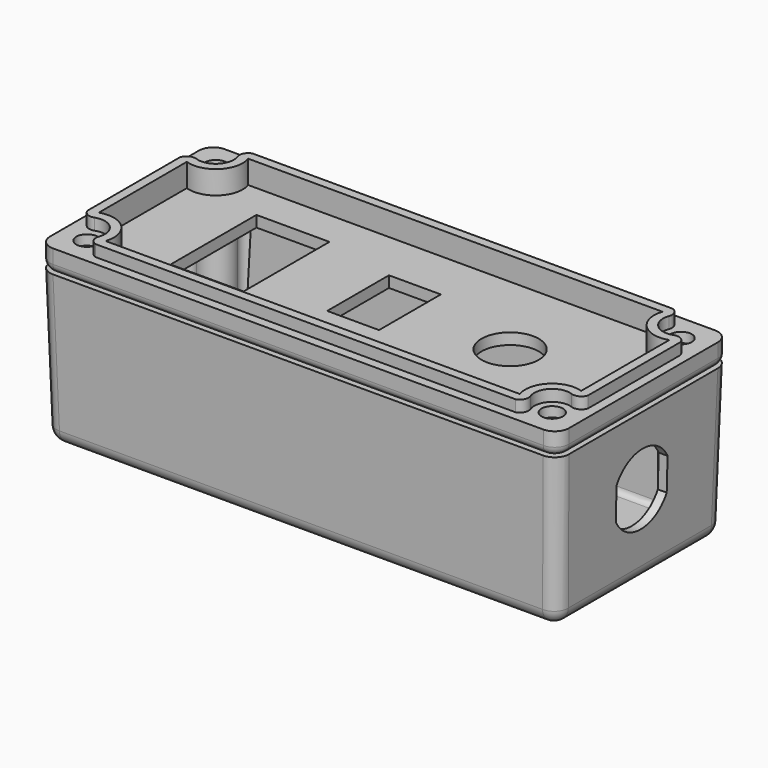
from build123d import *

# Parameters (mm, degrees)
F0_W            = 92.075
F0_H            = 38.1
F1_DEPTH        = 26.9748
F1_TAPER        = 1.5
F2_R            = 2.54
F3_T            = 1.5748
F6_DEPTH        = 23.0124
F8_D            = 2.7051
F8_DEPTH        = 12.7
F8_TIP          = 0.8126940303
F10_DEPTH       = 4.064
F13_DEPTH       = 2.032
F15_DEPTH       = 2.0828
F17_D           = 3.7973
F17_CSINK_D     = 7.7978
F17_CSINK_ANGLE = 82
F18_T1_DEPTH    = 86.995
F18_T3_DEPTH    = 33.02
F18_T6_ANGLE    = 90
F18_T8_ANGLE    = 90
F18_T10_ANGLE   = 90
F18_T12_ANGLE   = 90
F19_W           = 12.954
F19_H           = 19.05
F19_R           = 5.08
F19_W_2         = 9.2
F19_H_2         = 13.7
F20_DEPTH       = 6.097
F22_DEPTH       = 92.0760001
F24_D           = 2.7051
F24_DEPTH       = 12.7
F24_TIP         = 0.8126940303


# Not quite as in the source:
# - a fillet or chamfer that OpenCascade refuses, or shapes differently, is made with other operations: its cross-section is extruded or revolved along the edge and cut away or added
# - a shell that OpenCascade refuses in one call is made with other operations: the cavity is built on its own and cut out


with BuildPart() as f1:
    # F0 (on Top) → F1 (new body)
    with BuildSketch(Plane.XY):
        with Locations((46.0375, 19.05)):
            Rectangle(F0_W, F0_H)
    extrude(amount=-F1_DEPTH, taper=F1_TAPER)

    # F2
    f2_edges = [f1.edges().sort_by_distance(p)[0] for p in [
        (91.72182, 0.35318, -13.4874),
        (46.0375, 0.70636, -26.9748),
        (0.35318, 0.35318, -13.4874),
        (0.35318, 37.74682, -13.4874),
        (0.70636, 19.05, -26.9748),
        (91.36864, 19.05, -26.9748),
        (91.72182, 37.74682, -13.4874),
        (46.0375, 37.39364, -26.9748),
    ]]
    fillet(f2_edges, radius=F2_R)

    # F3: shell of thickness 1.5748, made by hand


with BuildPart() as f3_core1:
    # F3_t2: copy of F1
    add(f1.part)

    # the walls: a layer under each face that stays
    f3_faces = [f3_core1.faces().sort_by_distance(p)[0] for p in [
        (0.3207944219, 19.05, -12.2506447244),
        (1.0647429252, 37.0352570748, -12.2643990402),
        (1.0647429252, 1.0647429252, -12.2643990402),
        (1.4083306813, 19.05, -26.2542069363),
        (46.0375, 37.7792055781, -12.2506447244),
        (46.0375, 0.3207944219, -12.2506447244),
        (91.0102570748, 37.0352570748, -12.2643990402),
        (91.0102570748, 1.0647429252, -12.2643990402),
        (91.7542055781, 19.05, -12.2506447244),
        (1.9274510394, 36.1725489858, -26.2542069186),
        (1.418333, 1.9278747208, -25.7674590413),
        (46.0375, 19.05, -26.9748),
        (46.0375, 36.6916693187, -26.2542069363),
        (46.0375, 1.4083306813, -26.2542069363),
        (90.1471252549, 36.6816670172, -25.7674590413),
        (90.1475489611, 1.9274510396, -26.2542069358),
        (90.6666693187, 19.05, -26.2542069363),
    ]]
    thicken(f3_faces, amount=-F3_T, mode=Mode.SUBTRACT)


with BuildPart() as f1_1:
    add(f1.part)

    # what is left inside the walls is the cavity
    f3_cavity = [f3_core1.part.solids().sort_by_distance(p)[0] for p in [
        (50.224462, 29.168476, -0.015748),
    ]]
    add(f3_cavity, mode=Mode.SUBTRACT)

    # F5 (on offset) → F6 (join, through all)
    with BuildSketch(Plane.XY.offset(-2.3876)):
        with BuildLine():
            ThreePointArc((1.5753398296, 28.8697382874), (2.2451150935, 30.1585071832), (3.6847191374, 30.351028267))
            ThreePointArc((3.6847191374, 30.351028267), (7.0075640303, 31.0924359697), (7.748971733, 34.4152808626))
            ThreePointArc((7.748971733, 34.4152808626), (7.9414928168, 35.8548849065), (9.2302617126, 36.5246601704))
            Line((9.2302617126, 36.5246601704), (1.5753398296, 36.5246601704))
            Line((1.5753398296, 36.5246601704), (1.5753398296, 28.8697382874))
        make_face()
        with BuildLine():
            Line((90.4996601704, 28.8697382874), (90.4996601704, 36.5246601704))
            Line((90.4996601704, 36.5246601704), (82.8447382874, 36.5246601704))
            ThreePointArc((82.8447382874, 36.5246601704), (84.1335071832, 35.8548849065), (84.326028267, 34.4152808626))
            ThreePointArc((84.326028267, 34.4152808626), (85.0674359697, 31.0924359697), (88.3902808626, 30.351028267))
            ThreePointArc((88.3902808626, 30.351028267), (89.8298849065, 30.1585071832), (90.4996601704, 28.8697382874))
        make_face()
        with BuildLine():
            ThreePointArc((7.748971733, 3.6847191374), (7.0075640303, 7.0075640303), (3.6847191374, 7.748971733))
            ThreePointArc((3.6847191374, 7.748971733), (2.2451150935, 7.9414928168), (1.5753398296, 9.2302617126))
            Line((1.5753398296, 9.2302617126), (1.5753398296, 1.5753398296))
            Line((1.5753398296, 1.5753398296), (9.2302617126, 1.5753398296))
            ThreePointArc((9.2302617126, 1.5753398296), (7.9414928168, 2.2451150935), (7.748971733, 3.6847191374))
        make_face()
        with BuildLine():
            Line((90.4996601704, 1.5753398296), (90.4996601704, 9.2302617126))
            ThreePointArc((90.4996601704, 9.2302617126), (89.8298849065, 7.9414928168), (88.3902808626, 7.748971733))
            ThreePointArc((88.3902808626, 7.748971733), (85.0674359697, 7.0075640303), (84.326028267, 3.6847191374))
            ThreePointArc((84.326028267, 3.6847191374), (84.1335071832, 2.2451150935), (82.8447382874, 1.5753398296))
            Line((82.8447382874, 1.5753398296), (90.4996601704, 1.5753398296))
        make_face()
    extrude(amount=-F6_DEPTH)

    # F8
    with Locations(Plane.XY.offset(-2.3876)):
        with Locations((4.7625, 33.3375), (4.7625, 4.7625), (87.3125, 4.7625), (87.3125, 33.3375)):
            Hole(F8_D / 2, depth=F8_DEPTH)
            with Locations((0, 0, -(F8_DEPTH + F8_TIP / 2))):  # 118° drill point
                Cone(0, F8_D / 2, F8_TIP, mode=Mode.SUBTRACT)

    # F21 (on Right) → F22 (cut, through all)
    with BuildSketch(Plane.YZ):
        with BuildLine():
            Line((24.7015, -15.1459940556), (24.7015, -9.3552953931))
            ThreePointArc((24.7015, -9.3552953931), (19.05, -5.9006447244), (13.3985, -9.3552953931))
            Line((13.3985, -9.3552953931), (13.3985, -15.1459940556))
            ThreePointArc((13.3985, -15.1459940556), (19.05, -18.6006447244), (24.7015, -15.1459940556))
        make_face()
    extrude(amount=F22_DEPTH, mode=Mode.SUBTRACT)

    # F24
    with Locations(Plane(origin=(0, 0, -26.9748), x_dir=(1, 0, 0), z_dir=(0, 0, -1))):
        with Locations((14.2875, -19.05), (77.7875, -19.05)):
            Hole(F24_D / 2, depth=F24_DEPTH)
            with Locations((0, 0, -(F24_DEPTH + F24_TIP / 2))):  # 118° drill point
                Cone(0, F24_D / 2, F24_TIP, mode=Mode.SUBTRACT)


with BuildPart() as f10:
    # F9 (on Top) → F10 (new body)
    with BuildSketch(Plane.XY):
        with BuildLine():
            ThreePointArc((0, 2.54), (0.7439487758, 0.7439487758), (2.54, 0))
            Line((2.54, 0), (89.535, 0))
            ThreePointArc((89.535, 0), (91.3310512242, 0.7439487758), (92.075, 2.54))
            Line((92.075, 2.54), (92.075, 35.56))
            ThreePointArc((92.075, 35.56), (91.3310512242, 37.3560512242), (89.535, 38.1))
            Line((89.535, 38.1), (2.54, 38.1))
            ThreePointArc((2.54, 38.1), (0.7439487758, 37.3560512242), (0, 35.56))
            Line((0, 35.56), (0, 2.54))
        make_face()
    extrude(amount=F10_DEPTH)

    # F12 (on face) → F13 (join)
    with BuildSketch(Plane.XY.offset(4.064)):
        with BuildLine():
            Line((1.637861336, 29.3090659528), (1.637861336, 8.7909340472))
            ThreePointArc((1.637861336, 8.7909340472), (2.4357202816, 7.8268374185), (3.6847191374, 7.748971733))
            ThreePointArc((3.6847191374, 7.748971733), (7.0075640303, 7.0075640303), (7.748971733, 3.6847191374))
            ThreePointArc((7.748971733, 3.6847191374), (7.8268374185, 2.4357202816), (8.7909340472, 1.637861336))
            Line((8.7909340472, 1.637861336), (83.2840659528, 1.637861336))
            ThreePointArc((83.2840659528, 1.637861336), (84.2481625815, 2.4357202816), (84.326028267, 3.6847191374))
            ThreePointArc((84.326028267, 3.6847191374), (85.0674359697, 7.0075640303), (88.3902808626, 7.748971733))
            ThreePointArc((88.3902808626, 7.748971733), (89.6392797184, 7.8268374185), (90.437138664, 8.7909340472))
            Line((90.437138664, 8.7909340472), (90.437138664, 29.3090659528))
            ThreePointArc((90.437138664, 29.3090659528), (89.6392797184, 30.2731625815), (88.3902808626, 30.351028267))
            ThreePointArc((88.3902808626, 30.351028267), (85.0674359697, 31.0924359697), (84.326028267, 34.4152808626))
            ThreePointArc((84.326028267, 34.4152808626), (84.2481625815, 35.6642797184), (83.2840659528, 36.462138664))
            Line((83.2840659528, 36.462138664), (8.7909340472, 36.462138664))
            ThreePointArc((8.7909340472, 36.462138664), (7.8268374185, 35.6642797184), (7.748971733, 34.4152808626))
            ThreePointArc((7.748971733, 34.4152808626), (7.0075640303, 31.0924359697), (3.6847191374, 30.351028267))
            ThreePointArc((3.6847191374, 30.351028267), (2.4357202816, 30.2731625815), (1.637861336, 29.3090659528))
        make_face()
        with BuildLine():
            ThreePointArc((82.787168874, 34.861938664), (83.9359236985, 29.9609236985), (88.836938664, 28.812168874))
            Line((88.836938664, 28.812168874), (88.836938664, 9.287831126))
            ThreePointArc((88.836938664, 9.287831126), (83.9359236985, 8.1390763015), (82.787168874, 3.238061336))
            Line((82.787168874, 3.238061336), (9.287831126, 3.238061336))
            ThreePointArc((9.287831126, 3.238061336), (8.1390763015, 8.1390763015), (3.238061336, 9.287831126))
            Line((3.238061336, 9.287831126), (3.238061336, 28.812168874))
            ThreePointArc((3.238061336, 28.812168874), (8.1390763015, 29.9609236985), (9.287831126, 34.861938664))
            Line((9.287831126, 34.861938664), (82.787168874, 34.861938664))
        make_face(mode=Mode.SUBTRACT)
    extrude(amount=F13_DEPTH)

    # F14 (on face) → F15 (cut)
    with BuildSketch(Plane.XY.offset(4.064)):
        with BuildLine():
            ThreePointArc((9.287831126, 34.861938664), (8.1390763015, 29.9609236985), (3.238061336, 28.812168874))
            Line((3.238061336, 28.812168874), (3.238061336, 9.287831126))
            ThreePointArc((3.238061336, 9.287831126), (8.1390763015, 8.1390763015), (9.287831126, 3.238061336))
            Line((9.287831126, 3.238061336), (82.787168874, 3.238061336))
            ThreePointArc((82.787168874, 3.238061336), (83.9359236985, 8.1390763015), (88.836938664, 9.287831126))
            Line((88.836938664, 9.287831126), (88.836938664, 28.812168874))
            ThreePointArc((88.836938664, 28.812168874), (83.9359236985, 29.9609236985), (82.787168874, 34.861938664))
            Line((82.787168874, 34.861938664), (9.287831126, 34.861938664))
        make_face()
    extrude(amount=-F15_DEPTH, mode=Mode.SUBTRACT)

    # F17 (through all)
    with Locations(Plane(origin=(0, 0, 0), x_dir=(1, 0, 0), z_dir=(0, 0, -1))):
        with Locations((4.7625, -4.7625), (4.7625, -33.3375), (87.3125, -4.7625), (87.3125, -33.3375)):
            CounterSinkHole(F17_D / 2, F17_CSINK_D / 2, counter_sink_angle=F17_CSINK_ANGLE)

    # F18: fillet of radius 1.5748 on 4 edges, made by hand

    # F18_s2 → F18_t1 (cut)
    with BuildSketch(Plane.YZ.offset(2.54)):
        with BuildLine():
            ThreePointArc((1.5748, 0), (0.461248241, 0.461248241), (0, 1.5748))
            Line((0, 1.5748), (0, 0))
            Line((0, 0), (1.5748, 0))
        make_face()
        with BuildLine():
            ThreePointArc((36.5252, 0), (37.638751759, 0.461248241), (38.1, 1.5748))
            Line((38.1, 1.5748), (38.1, 0))
            Line((38.1, 0), (36.5252, 0))
        make_face()
    extrude(amount=F18_T1_DEPTH, mode=Mode.SUBTRACT)

    # F18_s4 → F18_t3 (cut)
    with BuildSketch(Plane.XZ.offset(-35.56)):
        with BuildLine():
            ThreePointArc((90.5002, 0), (91.613751759, 0.461248241), (92.075, 1.5748))
            Line((92.075, 1.5748), (92.075, 0))
            Line((92.075, 0), (90.5002, 0))
        make_face()
        with BuildLine():
            ThreePointArc((0, 1.5748), (0.461248241, 0.461248241), (1.5748, 0))
            Line((1.5748, 0), (0, 0))
            Line((0, 0), (0, 1.5748))
        make_face()
    extrude(amount=F18_T3_DEPTH, mode=Mode.SUBTRACT)

    # F18_s5 → F18_t6 (revolve, cut)
    with BuildSketch(Plane.YZ.offset(2.54)):
        with BuildLine():
            ThreePointArc((38.1, 1.5748), (37.638751759, 0.461248241), (36.5252, 0))
            Line((36.5252, 0), (38.1, 0))
            Line((38.1, 0), (38.1, 1.5748))
        make_face()
    revolve(axis=Axis((2.54, 35.56, 0), (0, 0, 1)), revolution_arc=F18_T6_ANGLE, mode=Mode.SUBTRACT)

    # F18_s7 → F18_t8 (revolve, cut)
    with BuildSketch(Plane.XZ.offset(-2.54)):
        with BuildLine():
            ThreePointArc((0, 1.5748), (0.461248241, 0.461248241), (1.5748, 0))
            Line((1.5748, 0), (0, 0))
            Line((0, 0), (0, 1.5748))
        make_face()
    revolve(axis=Axis((2.54, 2.54, 0), (0, 0, 1)), revolution_arc=F18_T8_ANGLE, mode=Mode.SUBTRACT)

    # F18_s9 → F18_t10 (revolve, cut)
    with BuildSketch(Plane.XZ.offset(-35.56)):
        with BuildLine():
            ThreePointArc((90.5002, 0), (91.613751759, 0.461248241), (92.075, 1.5748))
            Line((92.075, 1.5748), (92.075, 0))
            Line((92.075, 0), (90.5002, 0))
        make_face()
    revolve(axis=Axis((89.535, 35.56, 0), (0, 0, 1)), revolution_arc=F18_T10_ANGLE, mode=Mode.SUBTRACT)

    # F18_s11 → F18_t12 (revolve, cut)
    with BuildSketch(Plane.YZ.offset(89.535)):
        with BuildLine():
            ThreePointArc((1.5748, 0), (0.461248241, 0.461248241), (0, 1.5748))
            Line((0, 1.5748), (0, 0))
            Line((0, 0), (1.5748, 0))
        make_face()
    revolve(axis=Axis((89.535, 2.54, 0), (0, 0, 1)), revolution_arc=F18_T12_ANGLE, mode=Mode.SUBTRACT)

    # F19 (on face) → F20 (cut, through all)
    with BuildSketch(Plane(origin=(0, 0, 0), x_dir=(1, 0, 0), z_dir=(0, 0, -1))):
        with Locations((22.2605, -19.05)):
            Rectangle(F19_W, F19_H)
        with Locations((68.4175, -19.05)):
            Circle(F19_R)
        with Locations((46.0375, -19.05)):
            Rectangle(F19_W_2, F19_H_2)
    extrude(amount=-F20_DEPTH, mode=Mode.SUBTRACT)


solid = Compound([f1_1.part, f10.part])
